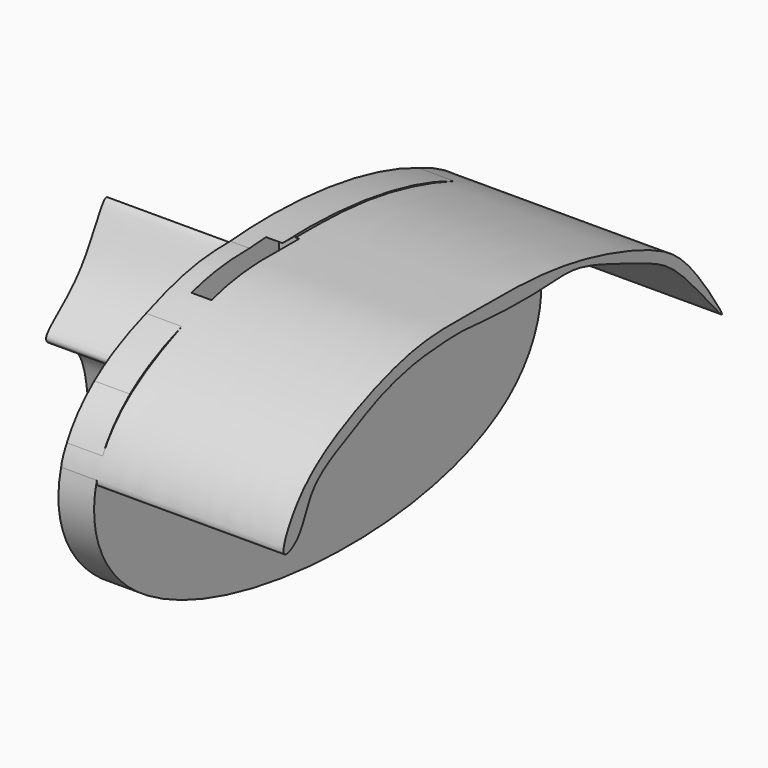
from build123d import *

# Parameters (mm, degrees)
F1_DEPTH = 12.7
F3_DEPTH = 63.754
F7_DEPTH = 79.248
F9_START = 6.858
F8_W     = 39.0965808183
F8_H     = 55.7831162587
F9_DEPTH = 7.112


# Not quite as in the source:
# - the program builds the solid bodies; features that only make, move or delete a surface that nothing else refers to are left out


with BuildPart() as f1:
    # F0 (on Right) → F1 (new body)
    with BuildSketch(Plane.YZ):
        with BuildLine():
            add(Edge.make_bspline(
                [(-52.2611625493, 26.7398431897), (-73.3956672979, 10.2636251119), (-74.4536998472, -60.3511227048), (143.3964165459, -74.3903950172), (129.9971801728, 53.8414934645), (-17.7469204758, 53.646751393), (-52.2611625493, 26.7398431897)],
                knots=[0, 0, 0, 0, 0.1869552725, 0.497788531, 0.6946879235, 1, 1, 1, 1], degree=3))
        make_face()
    extrude(amount=F1_DEPTH)

    # F2 (on Right) → F3 (join)
    with BuildSketch(Plane.YZ):
        with BuildLine():
            add(Edge.make_bspline(
                [(25.5373902619, -32.8582637012), (23.880955694, -32.295067065), (25.4080802802, -10.3710439907), (-3.0362550269, -6.0578005874), (23.3270062821, 7.0730743754), (34.0223532453, 39.8891350095), (36.9864422083, 8.3517150992), (58.7011474805, -4.0651674303), (36.328619379, -10.4823330589), (27.3733911611, -33.482513853), (25.5373902619, -32.8582637012)],
                knots=[0, 0, 0, 0, 0.1222534435, 0.2401597044, 0.3683803324, 0.5035913534, 0.6280396504, 0.7485566308, 0.864493632, 1, 1, 1, 1], degree=3))
        make_face()
    extrude(amount=-F3_DEPTH)

    # F6 (on Right) → F7 (join)
    with BuildSketch(Plane.YZ):
        with BuildLine():
            add(Edge.make_bspline(
                [(-66.6806325316, 3.9831637405), (-68.1510009104, 5.4628637765), (-60.7262480134, 22.0344349246), (-37.6633491867, 36.0594238534), (-7.7225924141, 46.526919325), (16.7983214039, 45.6961238978), (41.9901346554, 46.0565073437), (68.5924517125, 42.751604923), (99.7725099809, 33.0059588456), (114.4364954309, 22.3678209045), (136.4263232991, -11.609238688), (110.1235581516, 21.8387480307), (97.5813163687, 28.758126143), (82.8134428016, 34.2288002193), (63.5664977574, 42.1227067534), (48.3162389502, 40.0781843442), (23.7232568215, 40.6020476884), (13.012373402, 42.1994470025), (-0.2583700585, 41.2937364033), (-10.0703143091, 40.2996750588), (-24.8444008892, 36.3513858228), (-37.659544962, 29.3946065839), (-55.5846559231, 21.434082298), (-58.4799132075, 6.3925095019), (-65.7291863238, 3.0256792023), (-66.6806325316, 3.9831637405)],
                knots=[0, 0, 0, 0, 0.0390303418, 0.0930490502, 0.1489583673, 0.1982954424, 0.2479082612, 0.3004156206, 0.3561438377, 0.403017388, 0.4503255529, 0.5007370224, 0.5423457769, 0.5812202791, 0.6259249918, 0.6660022875, 0.7148914194, 0.7486792739, 0.7840288738, 0.8159156218, 0.8542020796, 0.8933323745, 0.9362323587, 0.9747442401, 1, 1, 1, 1], degree=3))
        make_face()
    extrude(amount=F7_DEPTH)

    # F8 (on Right) → F9 (cut)
    with BuildSketch(Plane.YZ.offset(F9_START)):
        with Locations((1.9685113803, 18.5587326996)):
            Rectangle(F8_W, F8_H)
    extrude(amount=F9_DEPTH, mode=Mode.SUBTRACT)


solid = f1.part
